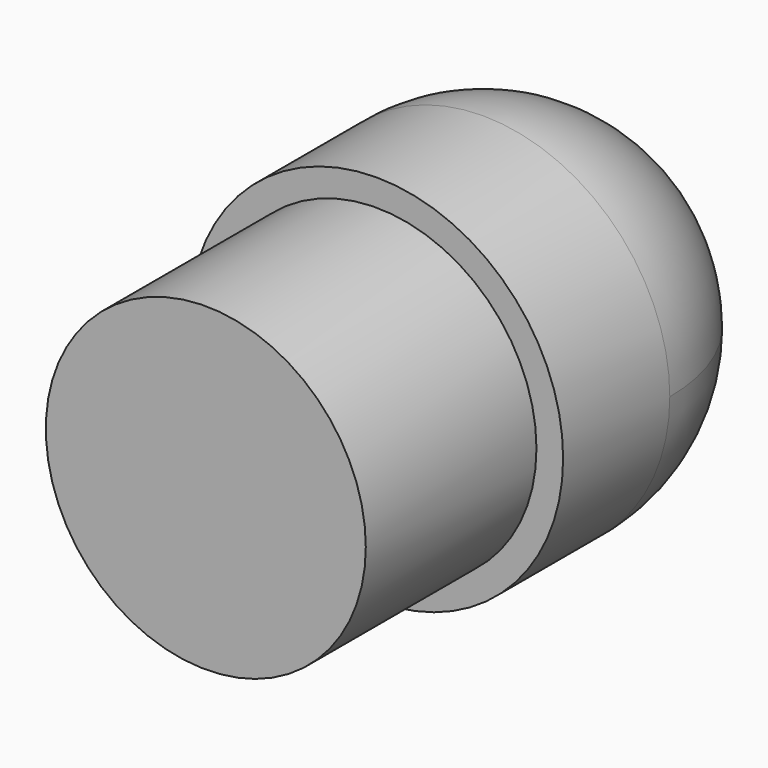
from build123d import *

# Parameters (mm, degrees)
F0_R     = 15
F1_DEPTH = 20
F2_R     = 17.5
F2_R_2   = 15
F3_DEPTH = 12.5


with BuildPart() as f1:
    # F0 (on Front) → F1 (new body)
    with BuildSketch(Plane.XZ):
        Circle(F0_R)
    extrude(amount=F1_DEPTH)

    # F2 (on face) → F3 (join)
    with BuildSketch(Plane(origin=(0, 0, 0), x_dir=(-1, 0, 0), z_dir=(0, 1, 0))):
        Circle(F2_R)
        Circle(F2_R_2, mode=Mode.SUBTRACT)
        Circle(F2_R_2)
    extrude(amount=F3_DEPTH)

    # F4 (on face) → F5 (revolve)
    with BuildSketch(Plane(origin=(0, 12.5, 0), x_dir=(-1, 0, 0), z_dir=(0, 1, 0))):
        with BuildLine():
            ThreePointArc((17.5, 0), (12.3743686708, 12.3743686708), (0, 17.5))
            Line((0, 17.5), (0, -17.5))
            ThreePointArc((0, -17.5), (12.3743686708, -12.3743686708), (17.5, 0))
        make_face()
    revolve(axis=Axis((0, 12.5, 0), (0, 0, -1)))


solid = f1.part
